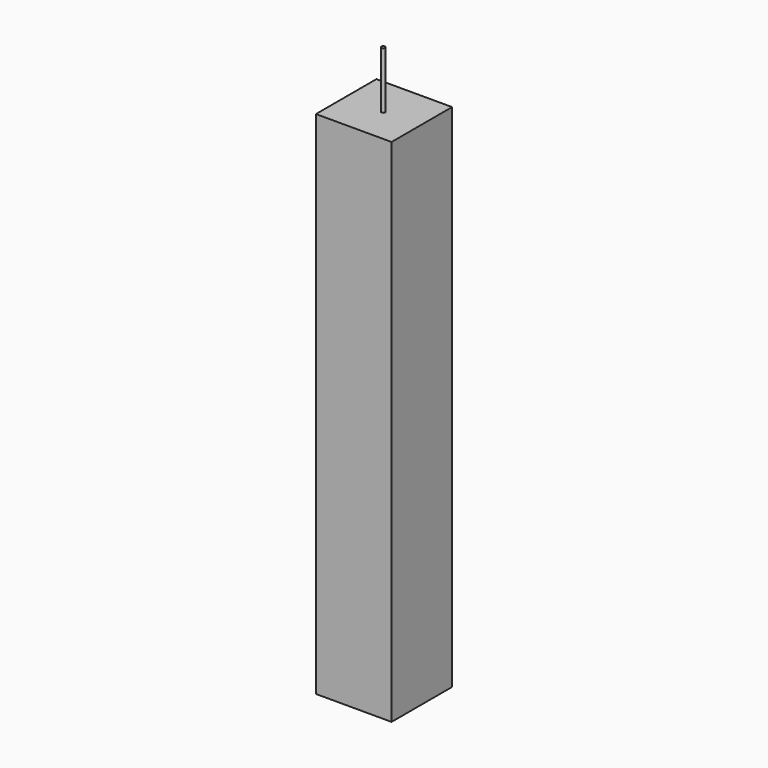
from build123d import *

# Parameters (mm, degrees)
F0_W     = 101.6
F0_H     = 101.6
F1_DEPTH = 685.8
F2_R     = 2.54
F3_DEPTH = 76.2


# Not quite as in the source:
# - a feature names something its author has since deleted; it is built from what else it names


with BuildPart() as f1:
    # F0 (on Top) → F1 (new body)
    with BuildSketch(Plane.XY):
        with Locations((5.0387959927, -3.5118889064)):
            Rectangle(F0_W, F0_H)
    extrude(amount=F1_DEPTH)

    # F2 (on face) → F3 (join)
    with BuildSketch(Plane.XY.offset(685.8)):
        with Locations((5.9797638096, -5.9394296259)):
            Circle(F2_R)
    extrude(amount=F3_DEPTH)


solid = f1.part
